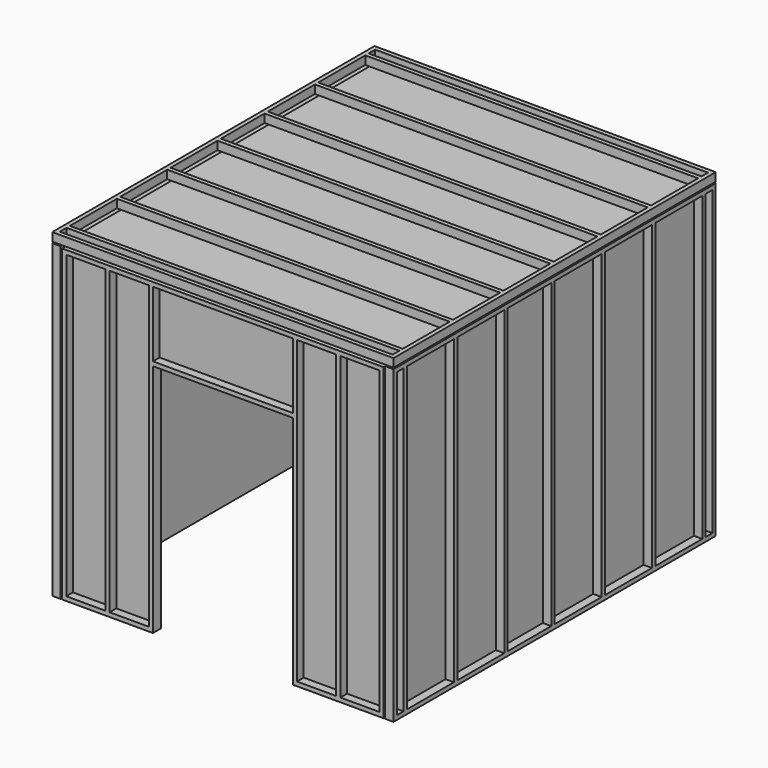
from build123d import *

# Parameters (mm, degrees)
F1_DEPTH  = 2819.4
F2_W      = 2946.4
F2_H      = 3505.2
F3_DEPTH  = 12.7
F4_W      = 1270
F4_H      = 2133.6
F5_DEPTH  = 3505.201
F6_W      = 38.1
F6_H      = 2730.5
F6_W_2    = 1270
F6_H_2    = 38.1
F7_DEPTH  = 76.2
F8_W      = 355.6
F8_H      = 2730.5
F8_W_2    = 1270
F8_H_2    = 596.9
F9_DEPTH  = 76.2
F10_W     = 38.1
F10_H     = 2743.2
F11_DEPTH = 76.2
F12_W     = 38.1
F12_H     = 2743.2
F13_DEPTH = 76.2
F14_W     = 3022.6
F14_H     = 76.2
F14_H_2   = 533.4
F14_H_3   = 532.384
F14_H_4   = 495.3
F14_H_5   = 74.168
F15_DEPTH = 76.2


with BuildPart() as f1:
    # F0 (on Top) → F1 (new body)
    with BuildSketch(Plane.XY):
        Polygon((153.5300910473, 2870.3572678566), (-993.4887962341, 2870.3572678566), (-993.4887962341, -634.8427321434), (882.2146654129, -634.8427321434), (913.4942889214, -634.8427321434), (1952.9112037659, -634.8427321434), (1952.9112037659, 2870.3572678566), (155.929601797, 2870.3572678566), align=None)
        Polygon((-980.7887962341, -622.1427321434), (-980.7887962341, 2857.6572678566), (149.7594565153, 2857.6572678566), (155.929601797, 2857.6572678566), (1940.2112037659, 2857.6572678566), (1940.2112037659, -622.1427321434), (1105.1017045975, -622.1427321434), (1102.0112037659, -622.1427321434), align=None, mode=Mode.SUBTRACT)
    extrude(amount=F1_DEPTH)

    # F4 (on face) → F5 (cut, through all)
    with BuildSketch(Plane.XZ.offset(634.8427321434)):
        with Locations((479.7112037659, 1066.8)):
            Rectangle(F4_W, F4_H)
    extrude(amount=-F5_DEPTH, mode=Mode.SUBTRACT)

    # F6 (on face) → F7 (join)
    with BuildSketch(Plane.XZ.offset(634.8427321434)):
        Polygon((-980.7887962341, 2806.7), (-980.7887962341, 2768.6), (-942.6887962341, 2768.6), (-587.0887962341, 2768.6), (-548.9887962341, 2768.6), (-193.3887962341, 2768.6), (-155.2887962341, 2768.6), (1114.7112037659, 2768.6), (1152.8112037659, 2768.6), (1508.4112037659, 2768.6), (1546.5112037659, 2768.6), (1902.1112037659, 2768.6), (1940.2112037659, 2768.6), (1940.2112037659, 2806.7), align=None)
        with Locations((-961.7387962341, 1403.35)):
            Rectangle(F6_W, F6_H)
        with Locations((-568.0387962341, 1403.35)):
            Rectangle(F6_W, F6_H)
        Polygon((-193.3887962341, 38.1), (-155.2887962341, 38.1), (-155.2887962341, 2133.6), (-155.2887962341, 2171.7), (-155.2887962341, 2768.6), (-193.3887962341, 2768.6), align=None)
        with Locations((479.7112037659, 2152.65)):
            Rectangle(F6_W_2, F6_H_2)
        Polygon((1114.7112037659, 2171.7), (1114.7112037659, 2133.6), (1114.7112037659, 38.1), (1152.8112037659, 38.1), (1152.8112037659, 2768.6), (1114.7112037659, 2768.6), align=None)
        with Locations((1527.4612037659, 1403.35)):
            Rectangle(F6_W, F6_H)
        with Locations((1921.1612037659, 1403.35)):
            Rectangle(F6_W, F6_H)
        Polygon((1152.8112037659, 38.1), (1114.7112037659, 38.1), (1114.7112037659, 0), (1940.2112037659, 0), (1940.2112037659, 38.1), (1902.1112037659, 38.1), (1546.5112037659, 38.1), (1508.4112037659, 38.1), align=None)
        Polygon((-980.7887962341, 38.1), (-980.7887962341, 0), (-155.2887962341, 0), (-155.2887962341, 38.1), (-193.3887962341, 38.1), (-548.9887962341, 38.1), (-587.0887962341, 38.1), (-942.6887962341, 38.1), align=None)
    extrude(amount=F7_DEPTH)

    # F8 (on face) → F9 (join)
    with BuildSketch(Plane(origin=(0, 2870.3572678566, 0), x_dir=(-1, 0, 0), z_dir=(0, 1, 0))):
        Polygon((-1940.2112037659, 0), (-1114.7112037659, 0), (-1114.7112037659, 2133.6), (155.2887962341, 2133.6), (155.2887962341, 0), (980.7887962341, 0), (980.7887962341, 2806.7), (-1940.2112037659, 2806.7), align=None)
        with Locations((-1724.3112037659, 1403.35)):
            Rectangle(F8_W, F8_H, mode=Mode.SUBTRACT)
        with Locations((-1330.6112037659, 1403.35)):
            Rectangle(F8_W, F8_H, mode=Mode.SUBTRACT)
        with Locations((371.1887962341, 1403.35)):
            Rectangle(F8_W, F8_H, mode=Mode.SUBTRACT)
        with Locations((764.8887962341, 1403.35)):
            Rectangle(F8_W, F8_H, mode=Mode.SUBTRACT)
        with Locations((-479.7112037659, 2470.15)):
            Rectangle(F8_W_2, F8_H_2, mode=Mode.SUBTRACT)
    extrude(amount=F9_DEPTH)

    # F10 (on face) → F11 (join)
    with BuildSketch(Plane.YZ.offset(1952.9112037659)):
        Polygon((2946.5572678566, 2819.4), (-711.0427321434, 2819.4), (-711.0427321434, 2781.3), (-672.9427321434, 2781.3), (-596.7427321434, 2781.3), (-558.6427321434, 2781.3), (-25.2427321434, 2781.3), (12.8572678566, 2781.3), (546.2572678566, 2781.3), (584.3572678566, 2781.3), (1079.6572678566, 2781.3), (1117.7572678566, 2781.3), (1651.1572678566, 2781.3), (1689.2572678566, 2781.3), (2222.6572678566, 2781.3), (2260.7572678566, 2781.3), (2794.1572678566, 2781.3), (2832.2572678566, 2781.3), (2908.4572678566, 2781.3), (2946.5572678566, 2781.3), align=None)
        with Locations((-691.9927321434, 1409.7)):
            Rectangle(F10_W, F10_H)
        with Locations((2927.5072678566, 1409.7)):
            Rectangle(F10_W, F10_H)
        Polygon((-672.9427321434, 38.1), (-711.0427321434, 38.1), (-711.0427321434, 0), (2946.5572678566, 0), (2946.5572678566, 38.1), (2908.4572678566, 38.1), (2832.2572678566, 38.1), (2794.1572678566, 38.1), (2260.7572678566, 38.1), (2222.6572678566, 38.1), (1689.2572678566, 38.1), (1651.1572678566, 38.1), (1117.7572678566, 38.1), (1079.6572678566, 38.1), (584.3572678566, 38.1), (546.2572678566, 38.1), (12.8572678566, 38.1), (-25.2427321434, 38.1), (-558.6427321434, 38.1), (-596.7427321434, 38.1), align=None)
        with Locations((-577.6927321434, 1409.7)):
            Rectangle(F10_W, F10_H)
        with Locations((-6.1927321434, 1409.7)):
            Rectangle(F10_W, F10_H)
        with Locations((565.3072678566, 1409.7)):
            Rectangle(F10_W, F10_H)
        with Locations((1098.7072678566, 1409.7)):
            Rectangle(F10_W, F10_H)
        with Locations((1670.2072678566, 1409.7)):
            Rectangle(F10_W, F10_H)
        with Locations((2241.7072678566, 1409.7)):
            Rectangle(F10_W, F10_H)
        with Locations((2813.2072678566, 1409.7)):
            Rectangle(F10_W, F10_H)
    extrude(amount=F11_DEPTH)

    # F12 (on face) → F13 (join)
    with BuildSketch(Plane(origin=(-993.4887962341, 0, 0), x_dir=(0, -1, 0), z_dir=(-1, 0, 0))):
        Polygon((711.0427321434, 2819.4), (-2946.5572678566, 2819.4), (-2946.5572678566, 2781.3), (-2908.4572678566, 2781.3), (-2832.2572678566, 2781.3), (-2794.1572678566, 2781.3), (-2260.7572678566, 2781.3), (-2222.6572678566, 2781.3), (-1689.2572678566, 2781.3), (-1651.1572678566, 2781.3), (-1155.8572678566, 2781.3), (-1117.7572678566, 2781.3), (-584.3572678566, 2781.3), (-546.2572678566, 2781.3), (-12.8572678566, 2781.3), (25.2427321434, 2781.3), (558.6427321434, 2781.3), (596.7427321434, 2781.3), (672.9427321434, 2781.3), (711.0427321434, 2781.3), align=None)
        with Locations((-2927.5072678566, 1409.7)):
            Rectangle(F12_W, F12_H)
        with Locations((691.9927321434, 1409.7)):
            Rectangle(F12_W, F12_H)
        Polygon((-2908.4572678566, 38.1), (-2946.5572678566, 38.1), (-2946.5572678566, 0), (711.0427321434, 0), (711.0427321434, 38.1), (672.9427321434, 38.1), (596.7427321434, 38.1), (558.6427321434, 38.1), (25.2427321434, 38.1), (-12.8572678566, 38.1), (-546.2572678566, 38.1), (-584.3572678566, 38.1), (-1117.7572678566, 38.1), (-1155.8572678566, 38.1), (-1651.1572678566, 38.1), (-1689.2572678566, 38.1), (-2222.6572678566, 38.1), (-2260.7572678566, 38.1), (-2794.1572678566, 38.1), (-2832.2572678566, 38.1), align=None)
        with Locations((-2813.2072678566, 1409.7)):
            Rectangle(F12_W, F12_H)
        with Locations((-2241.7072678566, 1409.7)):
            Rectangle(F12_W, F12_H)
        with Locations((-1670.2072678566, 1409.7)):
            Rectangle(F12_W, F12_H)
        with Locations((-1136.8072678566, 1409.7)):
            Rectangle(F12_W, F12_H)
        with Locations((-565.3072678566, 1409.7)):
            Rectangle(F12_W, F12_H)
        with Locations((6.1927321434, 1409.7)):
            Rectangle(F12_W, F12_H)
        with Locations((577.6927321434, 1409.7)):
            Rectangle(F12_W, F12_H)
    extrude(amount=F13_DEPTH)


with BuildPart() as f3:
    # F2 (on face) → F3 (new body)
    with BuildSketch(Plane.XY.offset(2819.4)):
        with Locations((479.7112037659, 1117.7572678566)):
            Rectangle(F2_W, F2_H)
    extrude(amount=F3_DEPTH)

    # F14 (on face) → F15 (join)
    with BuildSketch(Plane.XY.offset(2832.1)):
        Polygon((-1069.6887962341, -711.0427321434), (2029.1112037659, -711.0427321434), (2029.1112037659, -596.7427321434), (2029.1112037659, -558.6427321434), (2029.1112037659, -25.2427321434), (2029.1112037659, 12.8572678566), (2029.1112037659, 546.2572678566), (2029.1112037659, 584.3572678566), (2029.1112037659, 1116.7412678566), (2029.1112037659, 1155.8572678566), (2029.1112037659, 1651.1572678566), (2029.1112037659, 1689.2572678566), (2029.1112037659, 2222.6572678566), (2029.1112037659, 2260.7572678566), (2029.1112037659, 2794.1572678566), (2029.1112037659, 2832.2572678566), (2029.1112037659, 2946.5572678566), (-1069.6887962341, 2946.5572678566), (-1069.6887962341, 2832.2572678566), (-1069.6887962341, 2794.1572678566), (-1069.6887962341, 2260.7572678566), (-1069.6887962341, 2222.6572678566), (-1069.6887962341, 1689.2572678566), (-1069.6887962341, 1651.1572678566), (-1069.6887962341, 1155.8572678566), (-1069.6887962341, 1116.7412678566), (-1069.6887962341, 584.3572678566), (-1069.6887962341, 546.2572678566), (-1069.6887962341, 12.8572678566), (-1069.6887962341, -25.2427321434), (-1069.6887962341, -558.6427321434), (-1069.6887962341, -596.7427321434), align=None)
        with Locations((479.7112037659, -634.8427321434)):
            Rectangle(F14_W, F14_H, mode=Mode.SUBTRACT)
        with Locations((479.7112037659, -291.9427321434)):
            Rectangle(F14_W, F14_H_2, mode=Mode.SUBTRACT)
        with Locations((479.7112037659, 279.5572678566)):
            Rectangle(F14_W, F14_H_2, mode=Mode.SUBTRACT)
        with Locations((479.7112037659, 850.5492678566)):
            Rectangle(F14_W, F14_H_3, mode=Mode.SUBTRACT)
        with Locations((479.7112037659, 1403.5072678566)):
            Rectangle(F14_W, F14_H_4, mode=Mode.SUBTRACT)
        with Locations((479.7112037659, 1955.9572678566)):
            Rectangle(F14_W, F14_H_2, mode=Mode.SUBTRACT)
        with Locations((479.7112037659, 2527.4572678566)):
            Rectangle(F14_W, F14_H_2, mode=Mode.SUBTRACT)
        with Locations((479.7112037659, 2869.3412678566)):
            Rectangle(F14_W, F14_H_5, mode=Mode.SUBTRACT)
    extrude(amount=F15_DEPTH)


solid = Compound([f1.part, f3.part])
